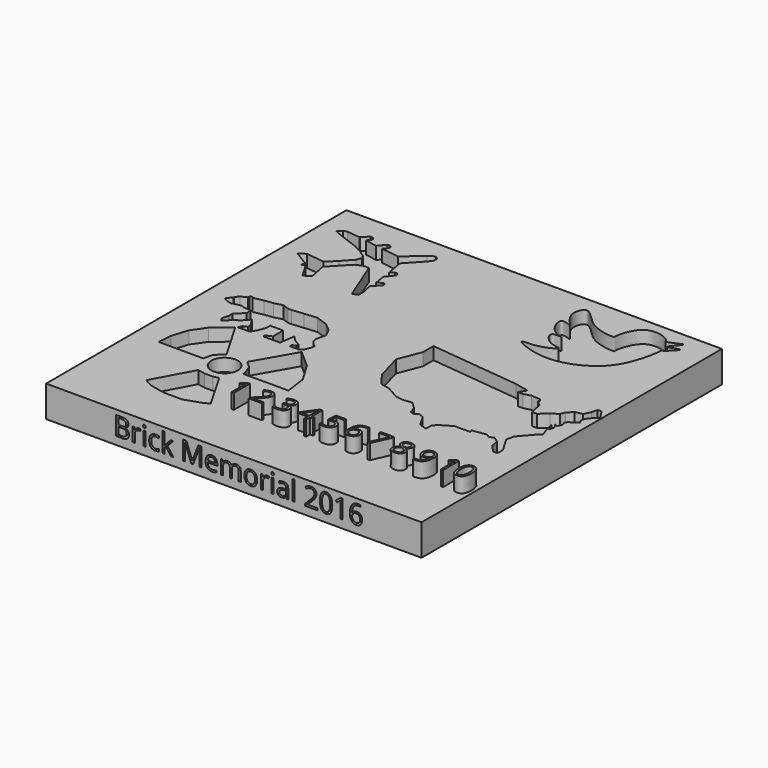
from build123d import *

# Parameters (mm, degrees)
F0_W         = 76.2
F0_H         = 76.2
F1_DEPTH     = 6.35
F3_DEPTH     = 2.54
F4_R         = 2.6882277056
F5_DEPTH     = 2.54
F6_TEXT_SIZE = 5.2878652544
F7_DEPTH     = 2.54
F8_TEXT_SIZE = 5.6723701871
F9_DEPTH     = 3.048
F11_DEPTH    = 2.54


# Not quite as in the source:
# - Text() gives the source's letters only with a copy of the font that has no kerning and outlines rounded to 1/6400 em; it was checked with that copy


with BuildPart() as f1:
    # F0 (on Top) → F1 (new body)
    with BuildSketch(Plane.XY):
        Rectangle(F0_W, F0_H)
    extrude(amount=F1_DEPTH)

    # F2 (on face) → F3 (cut)
    with BuildSketch(Plane.XY.offset(6.35)):
        Polygon((29.1530881077, 2.4021458812), (28.1402133405, 2.4021458812), (27.5937858969, 4.957952071), (26.5230343721, 5.8892657279), (26.7671439797, 6.0601425357), (26.3813771307, 6.6112377681), (24.5627630502, 6.7214565352), (23.1850259006, 6.3356901519), (22.1379455179, 6.3356901519), (22.9645874351, 7.6918248087), (20.1540030539, 8.3196321502), (1.8011641223, 10.3035746142), (1.8011641223, 7.6918248087), (0, 3.0221156776), (1.5417359537, -2.4691161234), (3.4874484409, -5.0201606937), (5.3899218328, -5.4525411688), (7.9888608307, -6.9330814295), (9.4526754692, -7.1628866717), (11.3121736795, -6.9330814295), (12.6427672803, -8.2017872483), (13.1688164547, -9.625214152), (13.9733618125, -9.872767143), (14.5303551108, -9.2848297209), (15.6544488646, -9.7613032325), (17.0368235558, -12.1007384732), (18.5840260237, -12.5958444551), (18.5840260237, -11.1105293036), (19.5542907689, -10.2412856822), (21.5546563268, -9.0592676156), (24.7998944764, -9.0592676156), (24.4943425059, -8.5421726108), (27.4030826986, -8.108955808), (28.1426586898, -8.6297875579), (28.9193429053, -8.1708440557), (30.1261618733, -8.9753894135), (30.4046571255, -10.4916477576), (31.7661948502, -12.0697952807), (32.6326303184, -12.0697952807), (32.7054481969, -10.7271157817), (30.8204200119, -7.5370245613), (31.1812199652, -5.9298304841), (33.2845523953, -3.4885213245), (34.2974252999, -2.4489918724), (33.8442996144, -1.302843797), (33.2845523953, 0.936142751), (33.9509174228, -0.6098242011), (34.2441163957, 0.4030507116), (33.72174854, 1.2870699129), (34.2441163957, 1.0694158264), (34.6439369023, 2.0289814565), (34.4040431082, 2.58872821), (34.7013784522, 3.184785283), (36.4031381905, 4.2946226895), (36.0033214092, 4.9076783471), (36.0033214092, 5.3608068265), (36.4297926426, 6.2137539499), (37.8158316016, 7.5997933745), (36.6163775325, 9.438960813), (35.8167402446, 9.438960813), (35.5235375464, 8.2395039499), (34.9104814231, 6.9067734294), (33.3911702037, 6.5869186074), (32.4049480259, 5.5740438402), (31.9784767926, 4.6144779772), (30.6990556419, 3.7881853059), align=None)
        Polygon((25.269200851, 5.0115818394), (26.5230343721, 5.8892657279), (25.9405020624, 4.0762000717), (25.269200851, 2.0922576077), align=None, mode=Mode.SUBTRACT)
        with BuildLine():
            add(Edge.make_bspline(
                [(11.6569008678, 20.2754884958), (11.6406454437, 20.0087809992), (15.8053606588, 18.1398607577), (21.5742803098, 18.3059575625), (26.6107238535, 20.9433946252), (29.4623787667, 24.5079972203), (30.908778947, 29.8391045483), (30.9354018343, 31.7977872334), (31.250061569, 31.6174806388), (34.8190521295, 35.0136554172), (29.0241390598, 31.9527326059), (34.380800112, 36.9117289409), (29.2587649479, 33.9303717088), (29.7190471855, 35.2663093413), (23.4687311139, 37.5909672568), (22.0462956154, 30.8284599407), (22.448684376, 30.4554078739), (16.7017596899, 30.6900272677), (13.087883438, 36.8768811446), (11.1997131934, 32.01402302), (15.4337277403, 28.6399825075), (11.2002551348, 30.8199213882), (12.9816179239, 25.7779949645), (17.0586064689, 25.1540405151), (12.664455592, 25.8757541622), (15.3845977099, 22.1510182761), (19.0980594306, 22.4620730889), (14.5342159235, 20.1352723286), (11.6706721491, 20.5014379341), (11.6569008678, 20.2754884958)],
                knots=[0, 0, 0, 0, 0.0426331114, 0.0972152109, 0.14729118, 0.1936929249, 0.2450656482, 0.2715044011, 0.2827111041, 0.3183230238, 0.3511142983, 0.3866432796, 0.4237106634, 0.4396683111, 0.4871367583, 0.5373310764, 0.5459848845, 0.5936099811, 0.644660133, 0.6818916146, 0.7210965091, 0.7496559301, 0.7908918475, 0.824014524, 0.8530723442, 0.8906501392, 0.922602032, 0.9638820517, 1, 1, 1, 1], degree=3))
        make_face()
        Polygon((-18.3084439486, 33.8336378336), (-21.7963326722, 30.8130141348), (-25.4098791629, 31.2975123525), (-24.885006249, 31.963698566), (-24.7235074639, 32.2665087879), (-24.7235074639, 32.609693706), (-25.0666923821, 32.8923203051), (-25.6117526442, 32.8923203051), (-26.1568129063, 32.2665087879), (-26.7826225609, 31.4791984856), (-29.2454883456, 31.9435112178), (-28.6196768284, 32.609693706), (-28.6196768284, 33.1143811345), (-29.0032383054, 33.3768166602), (-29.467549175, 33.3768166602), (-30.676741153, 32.2665087879), (-30.676741153, 32.1373380721), (-33.3543382585, 32.4429348111), (-34.0964980423, 32.2665087879), (-34.8677635193, 31.4791984856), (-33.1980958581, 30.7457242161), (-29.3041486293, 29.3208695948), (-27.6353135705, 28.4425355494), (-26.3080522418, 27.515405789), (-25.8889440447, 26.8280021846), (-26.3080522418, 25.7650334388), (-28.1496196985, 23.7588714808), (-29.8711825162, 22.026931867), (-33.6312912405, 22.5061625242), (-34.8677635193, 21.6398630291), (-31.7145138979, 19.7231248021), (-32.1872380204, 18.9454405366), (-31.2749892473, 19.2348212004), (-29.5478645712, 16.2114351988), (-28.1927859301, 16.985530785), (-28.9059206843, 20.6194464117), (-25.4394263029, 24.2571271956), (-24.1555385292, 24.8562749475), (-22.9572448879, 24.8562749475), (-19.4907505065, 16.2114351988), (-18.4651953023, 16.6226725909), (-18.4651953023, 17.966080457), (-18.8916027546, 19.7231248021), (-18.8916027546, 20.1200377196), (-17.8347826004, 21.1660359055), (-17.4795370549, 21.5804874897), (-17.4795370549, 22.0344122499), (-17.9334618151, 22.2909785807), (-18.8916027546, 21.6396953911), (-19.2557629198, 23.9290520549), (-18.3084439486, 25.0539947301), (-17.9334618151, 25.6658047438), (-18.1505568326, 26.1986721307), (-18.7426321208, 26.1986721307), (-19.4907505065, 25.6658047438), (-19.7053998709, 26.9611086696), (-20.0916491449, 29.1495136917), (-17.1155501157, 32.3326475918), (-16.4685696363, 33.2125388086), (-16.4685696363, 34.0924300253), (-17.1155501157, 34.5841310918), align=None)
        Polygon((25.9405020624, 4.0762000717), (26.5230343721, 5.8892657279), (25.269200851, 5.0115818394), (25.269200851, 2.0922576077), align=None)
    extrude(amount=-F3_DEPTH, mode=Mode.SUBTRACT)

    # F4 (on face) → F5 (cut)
    with BuildSketch(Plane.XY.offset(6.35)):
        Polygon((-23.6217454076, -13.9583060518), (-22.0393966883, -12.3759573326), (-26.7231483012, -4.3376288377), (-30.0144311041, -7.0592677221), (-31.8499542773, -9.7176125273), (-32.8626595438, -12.9456035793), (-33.1158339977, -15.7938301563), (-24.064803496, -15.7938301563), align=None)
        Polygon((-13.2415406406, -4.3376288377), (-17.8619977087, -12.3759573326), (-16.5800247341, -13.4982336313), (-15.8769395202, -15.2100948617), (-15.7732982188, -15.9837119281), (-6.5956781618, -15.9837119281), (-7.2286175564, -11.5531366318), (-9.6970805898, -7.4390312657), align=None)
        Polygon((-13.4373782203, -27.1354690194), (-17.8619977087, -19.4570142776), (-18.9843922853, -19.7042766958), (-20.6631775945, -19.7042766958), (-22.1600240479, -19.3846437408), (-26.4279711992, -27.2803455591), (-24.6411617845, -28.2461885363), (-21.5021707118, -28.8739874959), (-17.8619977087, -28.8739874959), (-14.5176039391, -27.7579364205), align=None)
        with Locations((-19.8715031147, -15.5885182321)):
            Circle(F4_R)
    extrude(amount=-F5_DEPTH, mode=Mode.SUBTRACT)

    # F6 (on face) → F7 (cut)
    with BuildSketch(Plane.XZ.offset(38.1)):
        with Locations((-24.3981726235, 1.6058408655)):
            Text('Brick Memorial 2016', F6_TEXT_SIZE, font='Open Sans', text_align=(TextAlign.LEFT, TextAlign.BOTTOM))
    extrude(amount=-F7_DEPTH, mode=Mode.SUBTRACT)

    # F8 (on face) → F9 (join)
    with BuildSketch(Plane.XY.offset(6.35)):
        with Locations((-11.197924614, -26.5783257782)):
            Text('1 2 3 4 5 6 7 8 9 10', F8_TEXT_SIZE, font='Open Sans', text_align=(TextAlign.LEFT, TextAlign.BOTTOM))
    extrude(amount=F9_DEPTH)

    # F10 (on face) → F11 (cut)
    with BuildSketch(Plane.XY.offset(6.35)):
        Polygon((-31.608235091, 5.4473513737), (-31.6288396716, 4.9996897578), (-32.809138298, 4.4202697463), (-33.3885587752, 3.7013594992), (-33.3456397057, 3.5082194954), (-34.2362299562, 2.6176290121), (-34.1825783253, 2.3386490066), (-33.0573543906, 1.8510486698), (-32.3993638158, 1.7396968324), (-30.6481029838, 2.1446128376), (-29.9293771386, 1.8510486698), (-28.5627860576, 1.8510486698), (-28.3855181187, 0.6525413482), (-30.0144311041, -0.8841495728), (-30.0144311041, -1.8830508925), (-30.3612630814, -3.1575111207), (-30.0144311041, -3.8808537647), (-29.0523581207, -3.0541764572), (-28.6734644324, -2.5030584075), (-27.6056732982, -1.9863855559), (-26.3656582683, -0.5741455825), (-25.2978671342, -2.1930548828), (-25.2978671342, -2.9163970612), (-26.090098545, -3.2608457841), (-26.4345481992, -4.0186331607), (-24.0234062076, -4.0186331607), (-23.3345087618, -2.8819523286), (-22.7833911777, -1.3663776917), (-22.7833911777, -0.4019212502), (-20.1311353594, -0.4019212502), (-20.1311353594, -2.985286992), (-21.4400403202, -3.5708497744), (-21.2602831202, -3.9726599608), (-17.926665023, -3.9726599608), (-17.4788814038, -0.8841495728), (-16.5833123028, -1.8486059271), (-15.239963308, -2.6408382691), (-15.239963308, -3.0886216555), (-15.9288607538, -3.467515111), (-15.9977506846, -3.9497436956), (-14.004371129, -3.9497436956), (-13.3875673637, -3.2497709617), (-12.9048516974, -2.0966157317), (-12.9048516974, -1.4529941836), (-13.5618811473, -0.9568691603), (-14.0445977449, -0.3400651622), (-14.2591381446, 0.5315056769), (-13.9105096459, 2.1137420554), (-13.7459468096, 2.4933810346), (-14.6690625697, 4.2934566736), (-16.2383578718, 5.5627408437), (-18.569227308, 6.3935448416), (-21.1770292372, 6.1627659015), (-23.5078949481, 5.9319869615), (-24.2694653571, 5.9319869615), (-25.5618281662, 6.416623015), (-27.1772816777, 5.9781428427), (-28.9542786777, 5.7473639026), (-30.9389773756, 5.3319619037), (-30.9985972431, 5.6168124189), align=None)
    extrude(amount=-F11_DEPTH, mode=Mode.SUBTRACT)


solid = f1.part
